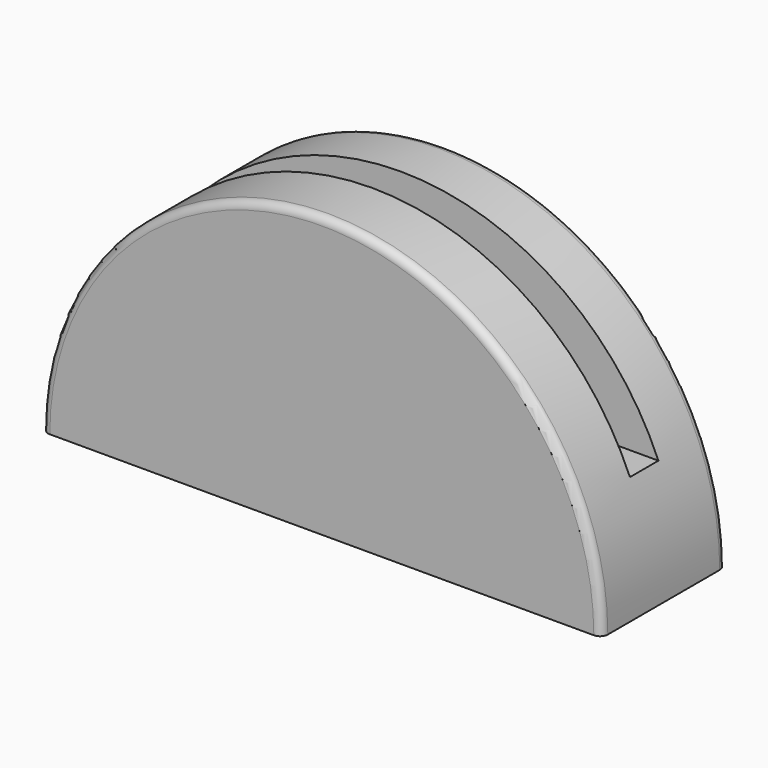
from build123d import *

# Parameters (mm, degrees)
F1_DEPTH      = 31.75
F2_W          = 14.5460739732
F2_H          = 83.8538557291
F3_DEPTH      = 114.301
F3_DEPTH_BACK = 114.301
F4_R          = 3.175
F5_T          = 2.54
F5_T3_DEPTH   = 215.6340543381


# Not quite as in the source:
# - a shell that OpenCascade refuses in one call is made with other operations: the cavity is built on its own and cut out


with BuildPart() as f1:
    # F0 (on Front) → F1 (new body, symmetric)
    with BuildSketch(Plane.XZ):
        with BuildLine():
            Line((-114.3, 0), (114.3, 0))
            ThreePointArc((114.3, 0), (0, 114.3), (-114.3, 0))
        make_face()
    extrude(amount=F1_DEPTH, both=True)

    # F2 (on Right) → F3 (cut, two sides)
    with BuildSketch(Plane.YZ) as f3_sk:
        with Locations((1.2597227469, 86.4380225539)):
            Rectangle(F2_W, F2_H)
    extrude(amount=-F3_DEPTH, mode=Mode.SUBTRACT)
    extrude(f3_sk.sketch, amount=F3_DEPTH_BACK, mode=Mode.SUBTRACT)

    # F4
    f4_edges = [f1.edges().sort_by_distance(p)[0] for p in [
        (0, 31.75, 114.3),
        (0, -31.75, 114.3),
    ]]
    fillet(f4_edges, radius=F4_R)

    # F5: shell of thickness 2.54, made by hand


with BuildPart() as f5_core1:
    # F5_t2: copy of F1
    add(f1.part)

    # the walls: a layer under each face that stays
    f5_faces = [f5_core1.faces().sort_by_distance(p)[0] for p in [
        (0, 31.75, 55.5625),
        (0, 30.8200640303, 113.3700640303),
        (98.9867036526, 19.05, 57.15),
        (0, -30.8200640303, 113.3700640303),
        (0, -31.75, 55.5625),
        (0, 8.5327597335, 79.4055473447),
        (0, 1.2597227469, 44.5110946894),
        (0, -6.0133142397, 79.4055473447),
    ]]
    thicken(f5_faces, amount=-F5_T, mode=Mode.SUBTRACT)

    # F5_s4 → F5_t3 (cut)
    with BuildSketch(Plane.YZ.offset(-107.8170271691)):
        Polygon((8.5073597335, 44.5364946894), (11.0727597335, 44.5110946894), (11.0727597335, 41.9710946894), (8.5327597335, 41.9710946894), align=None)
        Polygon((-5.9879142397, 44.5364946894), (-6.0133142397, 41.9710946894), (-8.5533142397, 41.9710946894), (-8.5533142397, 44.5110946894), align=None)
    extrude(amount=F5_T3_DEPTH, mode=Mode.SUBTRACT)


with BuildPart() as f1_1:
    add(f1.part)

    # what is left inside the walls is the cavity
    f5_cavity = [f5_core1.part.solids().sort_by_distance(p)[0] for p in [
        (0, 29.1846, 37.041667),
    ]]
    add(f5_cavity, mode=Mode.SUBTRACT)


solid = f1_1.part
